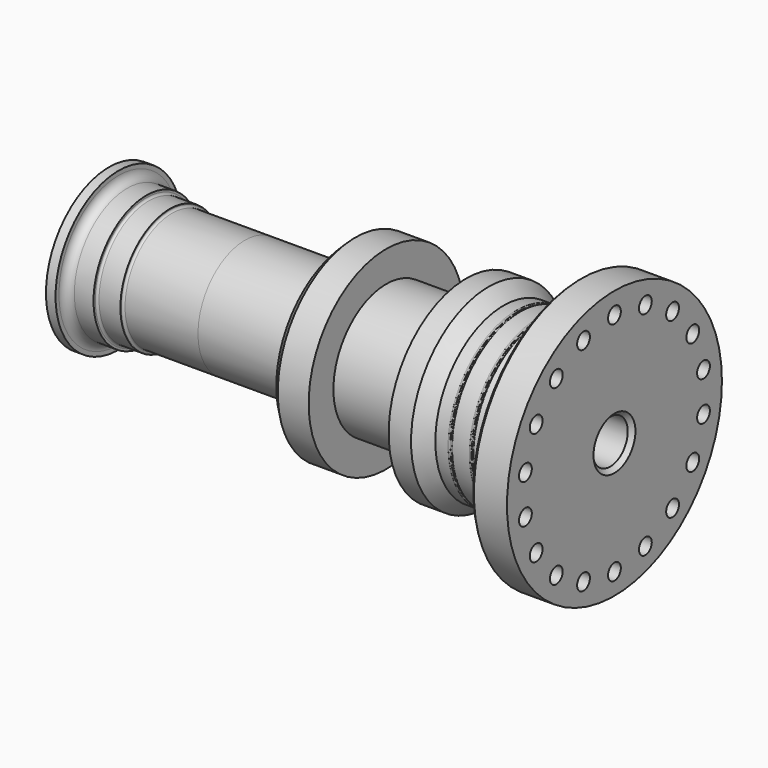
from build123d import *

# Parameters (mm, degrees)
F2_R             = 5
F3_R             = 40
F4_SIZE          = 15
F7_R             = 40
F8_SIZE          = 35
F11_R            = 40
F12_R            = 10
F13_R            = 37.5
F14_DEPTH        = 170
F14_COPIES_COUNT = 18
F15_SIZE         = 20


# Not quite as in the source:
# - a pattern or mirror of a feature is missing from the dataset's text; its kind, count and spacing are read off the source's solid


with BuildPart() as f1:
    # F0 (on Top) → F1 (revolve)
    with BuildSketch(Plane.XY):
        with BuildLine():
            Line((-1070, 102.87), (0, 102.87))
            Line((0, 102.87), (0, 630))
            Line((0, 630), (-170, 630))
            Line((-170, 630), (-170, 400))
            Line((-170, 400), (-342, 400))
            Line((-342, 400), (-350, 392))
            Line((-350, 392), (-358, 400))
            Line((-358, 400), (-442, 400))
            Line((-442, 400), (-450, 392))
            Line((-450, 392), (-458, 400))
            Line((-458, 400), (-520, 400))
            Line((-520, 400), (-590, 455))
            Line((-590, 455), (-695, 455))
            Line((-695, 455), (-695, 310))
            Line((-695, 310), (-1070, 310))
            Line((-1070, 310), (-1070, 240.87))
            ThreePointArc((-1070, 240.87), (-1083.9805777598, 238.2047342639), (-1096, 230.5828129211))
            Line((-1096, 230.5828129211), (-1096, 175.1571870789))
            ThreePointArc((-1096, 175.1571870789), (-1083.9805777598, 167.5352657361), (-1070, 164.87))
            Line((-1070, 164.87), (-1070, 102.87))
        make_face()
    revolve(axis=Axis((-650.086361788, 0, 0), (1, 0, 0)))

    # F2
    f2_edges = [f1.edges().sort_by_distance(p)[0] for p in [
        (-450, -392, 0),
        (-350, -392, 0),
        (-458, -400, 0),
        (-442, -400, 0),
        (-358, -400, 0),
        (-342, -400, 0),
    ]]
    fillet(f2_edges, radius=F2_R)

    # F3
    f3_edges = [f1.edges().sort_by_distance(p)[0] for p in [
        (-170, -400, 0),
    ]]
    fillet(f3_edges, radius=F3_R)

    # F4
    f4_edges = [f1.edges().sort_by_distance(p)[0] for p in [
        (-170, -630, 0),
    ]]
    chamfer(f4_edges, length=F4_SIZE)

    # F13 (on face) → F14 (cut, through all)
    with BuildSketch(Plane.YZ):
        with Locations((0, 530)):
            Circle(F13_R)
    f14 = extrude(amount=-F14_DEPTH, mode=Mode.SUBTRACT)

    # F14_copies: F14 ×18 about axis
    f14_copies_axis = Axis((0, 0, 0), (1, 0, 0))
    for i in range(1, F14_COPIES_COUNT):
        add(f14.rotate(f14_copies_axis, i * 360 / F14_COPIES_COUNT), mode=Mode.SUBTRACT)

    # F15
    f15_edges = [f1.edges().sort_by_distance(p)[0] for p in [
        (0, -102.87, 0),
    ]]
    chamfer(f15_edges, length=F15_SIZE)


with BuildPart() as f6:
    # F5 (on Top) → F6 (revolve)
    with BuildSketch(Plane.XY):
        with BuildLine():
            Line((-1733, 102.87), (-1070, 102.87))
            Line((-1070, 102.87), (-1070, 157.87))
            ThreePointArc((-1070, 157.87), (-1092.5250139353, 163.9133093395), (-1109, 180.4200556794))
            Line((-1109, 180.4200556794), (-1109, 225.3199443206))
            ThreePointArc((-1109, 225.3199443206), (-1092.5250139353, 241.8266906605), (-1070, 247.87))
            Line((-1070, 247.87), (-1070, 455))
            Line((-1070, 455), (-1250, 455))
            Line((-1250, 455), (-1250, 275))
            Line((-1250, 275), (-1733, 275))
            Line((-1733, 275), (-1733, 247.87))
            ThreePointArc((-1733, 247.87), (-1710.4749860647, 241.8266906605), (-1694, 225.3199443206))
            Line((-1694, 225.3199443206), (-1694, 180.4200556794))
            ThreePointArc((-1694, 180.4200556794), (-1710.4749860647, 163.9133093395), (-1733, 157.87))
            Line((-1733, 157.87), (-1733, 102.87))
        make_face()
    revolve(axis=Axis((-1474.7253394127, 0, 0), (-1, 0, 0)))

    # F7
    f7_edges = [f6.edges().sort_by_distance(p)[0] for p in [
        (-1250, -275, 0),
    ]]
    fillet(f7_edges, radius=F7_R)

    # F8
    f8_edges = [f6.edges().sort_by_distance(p)[0] for p in [
        (-1250, -455, 0),
    ]]
    chamfer(f8_edges, length=F8_SIZE)


with BuildPart() as f10:
    # F9 (on Top) → F10 (revolve)
    with BuildSketch(Plane.XY):
        with BuildLine():
            Line((-2370, 102.87), (-1733, 102.87))
            Line((-1733, 102.87), (-1733, 164.87))
            ThreePointArc((-1733, 164.87), (-1719.0194222402, 167.5352657361), (-1707, 175.1571870789))
            Line((-1707, 175.1571870789), (-1707, 230.5828129211))
            ThreePointArc((-1707, 230.5828129211), (-1719.0194222402, 238.2047342639), (-1733, 240.87))
            Line((-1733, 240.87), (-1733, 275))
            Line((-1733, 275), (-2085, 275))
            Line((-2085, 275), (-2085, 290))
            Line((-2085, 290), (-2195, 290))
            Line((-2195, 290), (-2195, 310))
            Line((-2195, 310), (-2325, 310))
            Line((-2325, 310), (-2325, 370))
            Line((-2325, 370), (-2370, 370))
            Line((-2370, 370), (-2370, 247.87))
            ThreePointArc((-2370, 247.87), (-2347.4749860647, 241.8266906605), (-2331, 225.3199443206))
            Line((-2331, 225.3199443206), (-2331, 180.4200556794))
            ThreePointArc((-2331, 180.4200556794), (-2347.4749860647, 163.9133093395), (-2370, 157.87))
            Line((-2370, 157.87), (-2370, 102.87))
        make_face()
    revolve(axis=Axis((-2225.577285956, 0, 0), (-1, 0, 0)))

    # F11
    f11_edges = [f10.edges().sort_by_distance(p)[0] for p in [
        (-2325, -310, 0),
    ]]
    fillet(f11_edges, radius=F11_R)

    # F12
    f12_edges = [f10.edges().sort_by_distance(p)[0] for p in [
        (-2195, -290, 0),
        (-2085, -275, 0),
    ]]
    fillet(f12_edges, radius=F12_R)


solid = Compound([f1.part, f6.part, f10.part])
